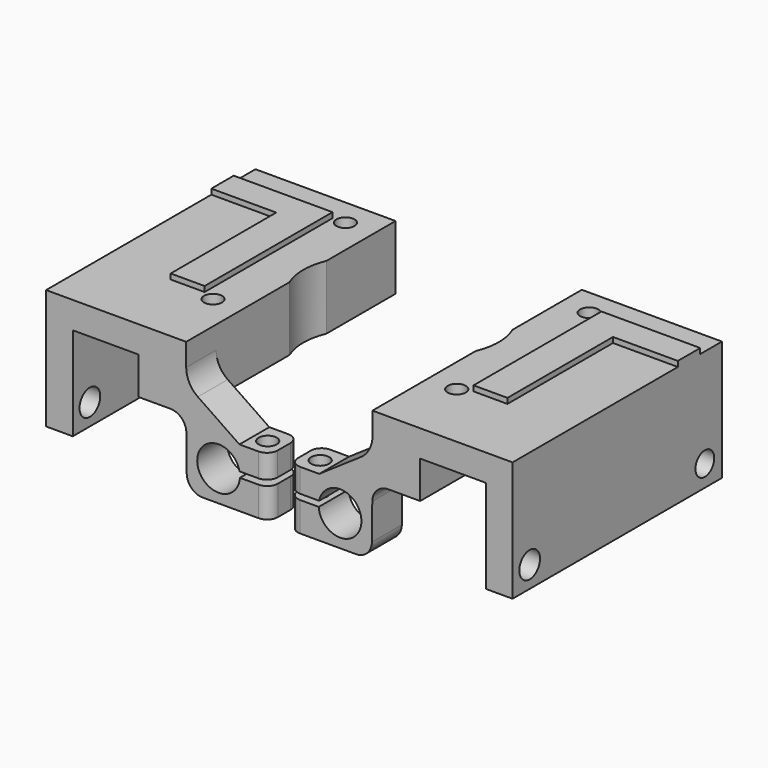
from build123d import *

# Parameters (mm, degrees)
F1_DEPTH      = 7
F2_DEPTH      = 42
F3_R          = 1.7
F3_R_2        = 11
F4_DEPTH      = 12.001
F5_R          = 4
F6_DEPTH      = 10
F7_DEPTH      = 12.001
F8_R          = 1.4
F9_DEPTH      = 10.9920075553
F8_R_2        = 1.7
F10_DEPTH     = 4.4348209087
F11_R         = 5
F12_R         = 3
F13_R         = 3
F14_R         = 2
F15_R         = 2.2
F15_R_2       = 2.4255023423
F16_DEPTH     = 6
F17_TEXT_SIZE = 41.9437823343
F18_DEPTH     = 1


# Not quite as in the source:
# - a feature names something its author has since deleted; it is built from what else it names
# - Text() gives the source's letters only with a copy of the font that has no kerning and outlines rounded to 1/6400 em; it was checked with that copy


with BuildPart() as f1:
    # F0 (on Front) → F1 (new body)
    with BuildSketch(Plane.XZ):
        Polygon((-18.6721007523, 29.8099789735), (-18.6721007523, 7.3259699669), (-13.6721007523, 7.3259699669), (-13.6721007523, 24.8099789735), (-1.3721007523, 24.8099789735), (-1.3721007523, 17.8099789735), (7.5637966118, 17.8099789735), (7.5637966118, 22.9406704692), (7.5637966118, 29.8099789735), align=None)
        Polygon((17.5301751077, 16.1394868046), (7.5637966118, 22.9406704692), (7.5637966118, 17.8099789735), (7.6940201178, 5.1484792493), (23.1186601057, 5.1484792493), (23.1186601057, 10.6682249423), (15.7860510706, 10.6682249423), (15.7860510706, 11.7046658959), (23.0896428882, 11.7046658959), (23.0896428882, 16.1394868046), align=None)
    extrude(amount=F1_DEPTH)

    # F0 (on Front) → F2 (join)
    with BuildSketch(Plane.XZ):
        Polygon((-18.6721007523, 29.8099789735), (-18.6721007523, 7.3259699669), (-13.6721007523, 7.3259699669), (-13.6721007523, 24.8099789735), (-1.3721007523, 24.8099789735), (-1.3721007523, 17.8099789735), (7.5637966118, 17.8099789735), (7.5637966118, 22.9406704692), (7.5637966118, 29.8099789735), align=None)
    extrude(amount=-F2_DEPTH)

    # F3 (on face) → F4 (cut, through all)
    with BuildSketch(Plane(origin=(0, 0, 17.8099789735), x_dir=(1, 0, 0), z_dir=(0, 0, -1))):
        with Locations((2.1850741468, -6)):
            Circle(F3_R)
        with Locations((2.1850741468, -37)):
            Circle(F3_R)
        with Locations((17.6850741468, -21.5)):
            Circle(F3_R_2)
    extrude(amount=-F4_DEPTH, mode=Mode.SUBTRACT)

    # F5 (on face) → F6 (cut)
    with BuildSketch(Plane.XZ.offset(7)):
        with Locations((13.6278992477, 10.8989789735)):
            Circle(F5_R)
    extrude(amount=-F6_DEPTH, mode=Mode.SUBTRACT)

    # F3 (on face) → F7 (cut, through all)
    with BuildSketch(Plane(origin=(0, 0, 17.8099789735), x_dir=(1, 0, 0), z_dir=(0, 0, -1))):
        with Locations((2.1850741468, -6)):
            Circle(F3_R)
        with Locations((2.1850741468, -37)):
            Circle(F3_R)
        with Locations((17.6850741468, -21.5)):
            Circle(F3_R_2)
    extrude(amount=-F7_DEPTH, mode=Mode.SUBTRACT)

    # F8 (on face) → F9 (cut, through all)
    with BuildSketch(Plane.XY.offset(16.1394868046)):
        with Locations((20.0896428882, -3.5767070949)):
            Circle(F8_R)
    extrude(amount=-F9_DEPTH, mode=Mode.SUBTRACT)

    # F8 (on face) → F10 (cut, through all)
    with BuildSketch(Plane.XY.offset(16.1394868046)):
        with Locations((20.0896428882, -3.5767070949)):
            Circle(F8_R_2)
        with Locations((20.0896428882, -3.5767070949)):
            Circle(F8_R, mode=Mode.SUBTRACT)
    extrude(amount=-F10_DEPTH, mode=Mode.SUBTRACT)

    # F11
    f11_edges = [f1.edges().sort_by_distance(p)[0] for p in [
        (7.563797, -3.5, 22.94067),
    ]]
    fillet(f11_edges, radius=F11_R)

    # F12
    f12_edges = [f1.edges().sort_by_distance(p)[0] for p in [
        (7.563797, -3.5, 17.809979),
    ]]
    fillet(f12_edges, radius=F12_R)

    # F13
    f13_edges = [f1.edges().sort_by_distance(p)[0] for p in [
        (7.69402, -3.5, 5.148479),
    ]]
    fillet(f13_edges, radius=F13_R)

    # F14
    f14_edges = [f1.edges().sort_by_distance(p)[0] for p in [
        (23.089643, -7, 13.922076),
        (23.11866, -7, 7.908352),
        (23.089643, 0, 13.922076),
        (23.11866, 0, 7.908352),
    ]]
    fillet(f14_edges, radius=F14_R)

    # F15 (on face) → F16 (cut)
    with BuildSketch(Plane(origin=(-18.6721007523, 0, 0), x_dir=(0, -1, 0), z_dir=(-1, 0, 0))):
        with Locations((-38, 11.3259699669)):
            Circle(F15_R)
        with Locations((3, 11.3259699669)):
            Circle(F15_R_2)
    extrude(amount=-F16_DEPTH, mode=Mode.SUBTRACT)

    # F17 (on face) → F18 (join)
    with BuildSketch(Plane.XY.offset(29.8099789735)):
        with Locations(Location((3.5908724648, 36.9253193088), (0, 0, 180))):
            Text('L', F17_TEXT_SIZE, font='Open Sans', font_style=FontStyle.BOLD, text_align=(TextAlign.LEFT, TextAlign.BOTTOM))
    extrude(amount=F18_DEPTH)


with BuildPart() as f19_1:
    # F19: instance of F1
    add(f1.part.mirror(Plane.YZ))


with BuildPart() as f19_1_1:
    # F20: moved
    add(f19_1.part.moved(Location((50, 0, 0))))


solid = Compound([f1.part, f19_1_1.part])
